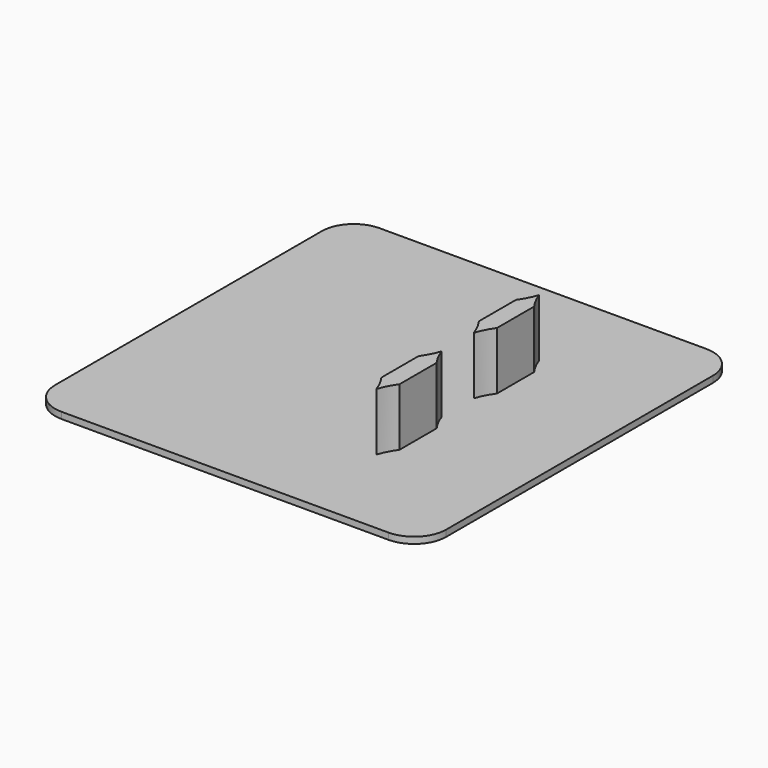
from build123d import *

# Parameters (mm, degrees)
F0_W     = 23
F0_H     = 62
F0_W_2   = 38
F1_DEPTH = 1
F2_DEPTH = 10
F3_R     = 5


# Not quite as in the source:
# - a feature names something its author has since deleted; it is built from what else it names


with BuildPart() as f1:
    # F0 (on Top) → F1 (new body)
    with BuildSketch(Plane.XY):
        with Locations((-21, 19)):
            Rectangle(F0_W, F0_H)
        with Locations((9.5, 19)):
            Rectangle(F0_W_2, F0_H)
        with BuildLine():
            ThreePointArc((9.5, 15.8775010008), (10.0985618966, 14.4432029131), (10.9121369044, 13.1189736826))
            Line((10.9121369044, 13.1189736826), (10.9121369044, 5.8810263174))
            ThreePointArc((10.9121369044, 5.8810263174), (10.0985618966, 4.5567970869), (9.5, 3.1224989992))
            ThreePointArc((9.5, 3.1224989992), (8.9014381034, 4.5567970869), (8.0878630956, 5.8810263174))
            Line((8.0878630956, 5.8810263174), (8.0878630956, 13.1189736826))
            ThreePointArc((8.0878630956, 13.1189736826), (8.9014381034, 14.4432029131), (9.5, 15.8775010008))
        make_face(mode=Mode.SUBTRACT)
        with BuildLine():
            Line((8.0878630956, 24.8810263174), (8.0878630956, 32.1189736826))
            ThreePointArc((8.0878630956, 32.1189736826), (8.9014381034, 33.4432029131), (9.5, 34.8775010008))
            ThreePointArc((9.5, 34.8775010008), (10.0985618966, 33.4432029131), (10.9121369044, 32.1189736826))
            Line((10.9121369044, 32.1189736826), (10.9121369044, 24.8810263174))
            ThreePointArc((10.9121369044, 24.8810263174), (10.0985618966, 23.5567970869), (9.5, 22.1224989992))
            ThreePointArc((9.5, 22.1224989992), (8.9014381034, 23.5567970869), (8.0878630956, 24.8810263174))
        make_face(mode=Mode.SUBTRACT)
    extrude(amount=F1_DEPTH)

    # F0 (on Top) → F2 (join)
    with BuildSketch(Plane.XY):
        with BuildLine():
            ThreePointArc((9.5, 34.8775010008), (8.9014381034, 33.4432029131), (8.0878630956, 32.1189736826))
            Line((8.0878630956, 32.1189736826), (8.0878630956, 24.8810263174))
            ThreePointArc((8.0878630956, 24.8810263174), (8.9014381034, 23.5567970869), (9.5, 22.1224989992))
            ThreePointArc((9.5, 22.1224989992), (10.0985618966, 23.5567970869), (10.9121369044, 24.8810263174))
            Line((10.9121369044, 24.8810263174), (10.9121369044, 32.1189736826))
            ThreePointArc((10.9121369044, 32.1189736826), (10.0985618966, 33.4432029131), (9.5, 34.8775010008))
        make_face()
        with BuildLine():
            Line((10.9121369044, 5.8810263174), (10.9121369044, 13.1189736826))
            ThreePointArc((10.9121369044, 13.1189736826), (10.0985618966, 14.4432029131), (9.5, 15.8775010008))
            ThreePointArc((9.5, 15.8775010008), (8.9014381034, 14.4432029131), (8.0878630956, 13.1189736826))
            Line((8.0878630956, 13.1189736826), (8.0878630956, 5.8810263174))
            ThreePointArc((8.0878630956, 5.8810263174), (8.9014381034, 4.5567970869), (9.5, 3.1224989992))
            ThreePointArc((9.5, 3.1224989992), (10.0985618966, 4.5567970869), (10.9121369044, 5.8810263174))
        make_face()
    extrude(amount=F2_DEPTH)

    # F3
    f3_edges = [f1.edges().sort_by_distance(p)[0] for p in [
        (-32.5, 50, 0.5),
        (28.5, 50, 0.5),
        (28.5, -12, 0.5),
        (-32.5, -12, 0.5),
    ]]
    fillet(f3_edges, radius=F3_R)


solid = f1.part
